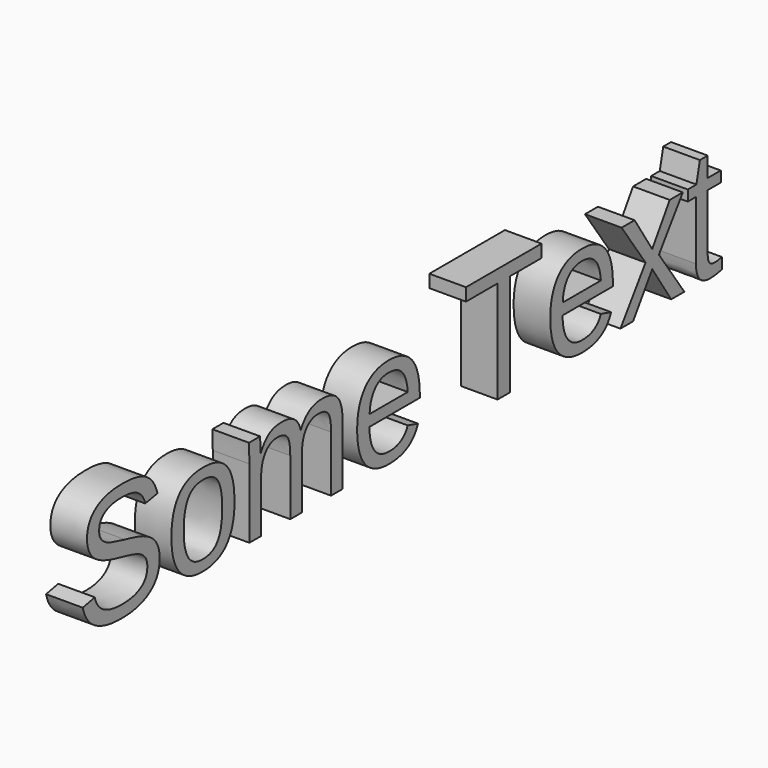
from build123d import *

# Parameters (mm, degrees)
F0_TEXT_SIZE = 115.8500193722
F1_DEPTH     = 25.4


# Not quite as in the source:
# - Text() gives the source's letters only with a copy of the font that has no kerning and outlines rounded to 1/6400 em; it was checked with that copy


with BuildPart() as f1:
    # F0 (on Right) → F1 (new body)
    with BuildSketch(Plane.YZ):
        with Locations((-567.2849620476, 0)):
            Text('Some Text', F0_TEXT_SIZE, font='Arimo', text_align=(TextAlign.LEFT, TextAlign.BOTTOM))
    extrude(amount=F1_DEPTH)


solid = f1.part
